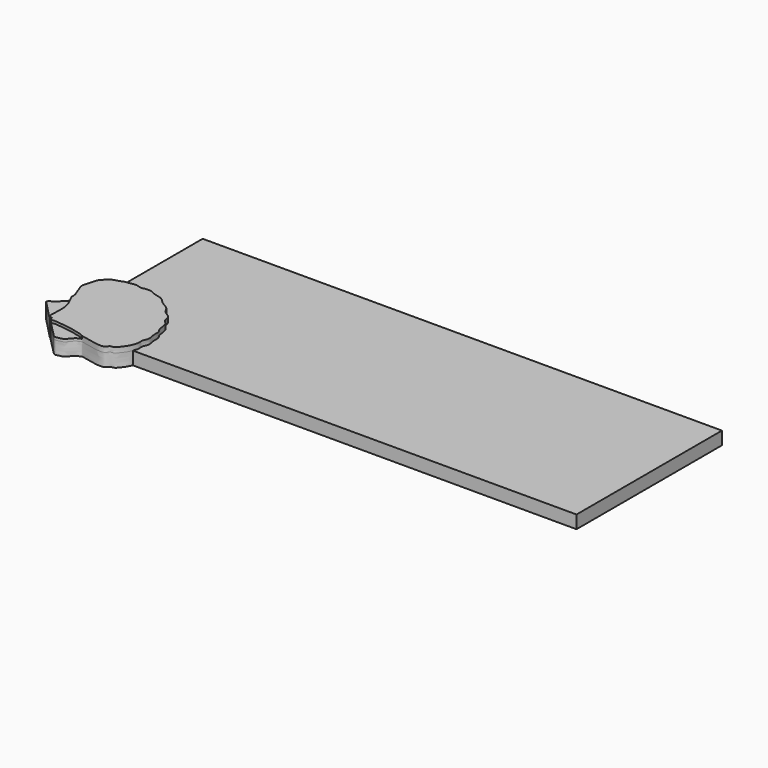
from build123d import *

# Parameters (mm, degrees)
F0_W          = 508
F0_H          = 177.8
F1_DEPTH      = 12.7
F4_DEPTH      = 12.7
F4_DEPTH_BACK = 5.08
F6_DEPTH      = 2.54


# Not quite as in the source:
# - the dataset's text gives a spline's control points without its knots; the knots are read off the source's solid


with BuildPart() as f1:
    # F0 (on Top) → F1 (new body)
    with BuildSketch(Plane.XY):
        Rectangle(F0_W, F0_H)
    extrude(amount=F1_DEPTH)

    # F3 (on face) → F4 (join, two sides)
    with BuildSketch(Plane.XY.offset(12.7)) as f4_sk:
        with BuildLine():
            add(Edge.make_bspline(
                [(-240.4387295246, -110.2688536048), (-239.7051986407, -111.0748850486), (-238.2641163582, -112.6584006965), (-235.2912335904, -111.9026221808), (-229.2381718402, -110.8419305219), (-227.0993916138, -106.6789146068), (-222.6995516224, -102.782071218), (-221.1790633511, -102.9183063508), (-219.8400801696, -101.7005143284), (-217.8203972939, -101.9296627609), (-212.4394677475, -103.1160593004), (-207.0370178023, -104.5088153919), (-200.4786957961, -105.5683418099), (-194.0950272547, -105.3397084837), (-192.7559850243, -101.0478482604), (-188.6782371307, -101.6121758975), (-185.4442125231, -97.7577508085), (-181.2489709308, -92.380579388), (-177.7257971457, -83.1360845172), (-179.4681627126, -79.5104890567), (-175.7040088945, -73.862192969), (-178.121500562, -67.4594844687), (-177.3641942685, -59.6556343554), (-180.867811307, -56.7481958192), (-180.8908481757, -45.5107362161), (-187.1323683475, -42.8995132365), (-186.6137909952, -35.0104892079), (-194.717327854, -32.3412016897), (-197.2445361966, -25.1829254152), (-202.7202510362, -22.4063482373), (-206.5360488835, -20.2143526951), (-210.1285132016, -15.4036668975), (-216.1747342712, -14.0173374922), (-220.3348552455, -13.0048669516), (-224.1354746673, -10.4978803172), (-230.6992753238, -10.6092105052), (-234.6813738561, -12.0408539375), (-239.0556379416, -9.5867149313), (-244.5594469356, -10.7151825488), (-250.4291116751, -11.378726385), (-254.5279405885, -13.5734994705), (-259.1780728115, -14.1353279262), (-262.2182152332, -16.8634259737), (-265.2208806455, -19.2320371154), (-267.9782545654, -22.4203833041), (-269.8411298683, -30.0636295196), (-271.9655718456, -36.5658221469), (-270.5631511784, -40.7346843912), (-267.4014672455, -48.4164619197), (-265.7871314271, -53.1938772949), (-266.4945228112, -60.0536176297), (-271.4618335405, -63.5192155045), (-274.9769319168, -66.9757623423), (-277.1950158231, -68.185338466), (-278.0953961719, -68.9306411766), (-278.5488670213, -69.1101614183), (-280.0349268792, -70.7807233404), (-278.5779237747, -71.630641818)],
                knots=[0, 0, 0, 0, 0.0142616055, 0.0282525416, 0.0481365155, 0.0663565385, 0.0858116795, 0.0955478407, 0.1057937238, 0.1172046473, 0.1365142573, 0.1565422226, 0.178296581, 0.1981966978, 0.2136916402, 0.228771452, 0.2464797559, 0.2689662054, 0.2943920012, 0.3101317365, 0.3301173561, 0.3518345571, 0.374113099, 0.3911763961, 0.4175369934, 0.4374585861, 0.4583521238, 0.4809459072, 0.5031937122, 0.5231432246, 0.5405283668, 0.5604126612, 0.5807938726, 0.5978739122, 0.6153247399, 0.6362499129, 0.6530397121, 0.6706356332, 0.6902034801, 0.7103871671, 0.7282286999, 0.745824621, 0.7623756412, 0.7784260605, 0.7951420444, 0.8185487682, 0.839965304, 0.8571701798, 0.8808429325, 0.8999737296, 0.9206064213, 0.9408137908, 0.9593472467, 0.9723775492, 0.9806544811, 0.9871724167, 1, 1, 1, 1], degree=3))
            Line((-278.5779237747, -71.630641818), (-258.092045784, -92.7531272173))
            Line((-258.092045784, -92.7531272173), (-255.9503316879, -92.7531272173))
            Line((-255.9503316879, -92.7531272173), (-255.9503316879, -94.6271494031))
            Line((-255.9503316879, -94.6271494031), (-240.4387295246, -110.2688536048))
        make_face()
    extrude(amount=-F4_DEPTH)
    extrude(f4_sk.sketch, amount=F4_DEPTH_BACK)

    # F5 (on face) → F6 (cut)
    with BuildSketch(Plane.XY.offset(17.78)):
        with BuildLine():
            add(Edge.make_bspline(
                [(-266.2298315407, -56.2032756853), (-265.7307978524, -57.2547741774), (-264.6827688199, -59.4787429503), (-262.2987003092, -63.5211859219), (-259.1637582398, -71.8378540614), (-259.4355894938, -81.0050752088), (-259.5171876554, -86.8522617588), (-259.8938502675, -89.0001691199), (-259.386488254, -90.2386261239), (-259.5751738001, -91.2239103647)],
                knots=[0, 0, 0, 0, 0.1218544331, 0.2618023507, 0.4550906777, 0.6563755288, 0.8112074375, 0.9021679838, 1, 1, 1, 1], degree=3))
            add(Edge.make_bspline(
                [(-266.2298315407, -56.2032756853), (-266.3796394264, -57.3738886427), (-267.2655118058, -60.5915219338), (-271.4618335405, -63.5192155045), (-274.9769319168, -66.9757623423), (-277.1950158231, -68.185338466), (-278.0953961719, -68.9306411766), (-278.5488670213, -69.1101614183), (-280.0349268792, -70.7807233404), (-278.5779237747, -71.630641818)],
                knots=[0.9091892449, 0.9091892449, 0.9091892449, 0.9091892449, 0.9206064213, 0.9408137908, 0.9593472467, 0.9723775492, 0.9806544811, 0.9871724167, 1, 1, 1, 1], degree=3))
            Line((-278.5779237747, -71.6306418181), (-259.5751738001, -91.2239103647))
        make_face()
        with BuildLine():
            add(Edge.make_bspline(
                [(-240.4387295246, -110.2688536048), (-239.7051986407, -111.0748850486), (-238.2641163582, -112.6584006965), (-235.2912335904, -111.9026221808), (-229.2381718402, -110.8419305219), (-227.0993916138, -106.6789146068), (-222.6995516224, -102.782071218), (-221.1790633511, -102.9183063509), (-220.2588870417, -102.0814150558), (-219.7109604479, -101.9094062854), (-219.6359576877, -101.890949453)],
                knots=[0, 0, 0, 0, 0.0142616055, 0.0282525416, 0.0481365155, 0.0663565385, 0.0858116795, 0.0955478407, 0.1057937238, 0.1073855615, 0.1073855615, 0.1073855615, 0.1073855615], degree=3))
            add(Edge.make_bspline(
                [(-219.6359576877, -101.890949453), (-220.3852001837, -101.2988761624), (-222.0968561153, -99.9304522565), (-227.2786685857, -99.2122646483), (-231.4429206973, -97.8065637376), (-238.2050623491, -96.7174296376), (-243.1780188905, -95.9940477016), (-251.3919772148, -95.0017124444), (-253.6224491485, -95.8020710086), (-254.480018374, -96.1097948254)],
                knots=[0, 0, 0, 0, 0.1113315842, 0.2544970345, 0.3921545206, 0.5556763146, 0.7058384241, 0.8868720946, 1, 1, 1, 1], degree=3))
            Line((-254.480018374, -96.1097948254), (-240.4387295246, -110.2688536048))
        make_face()
    extrude(amount=-F6_DEPTH, mode=Mode.SUBTRACT)


solid = f1.part
